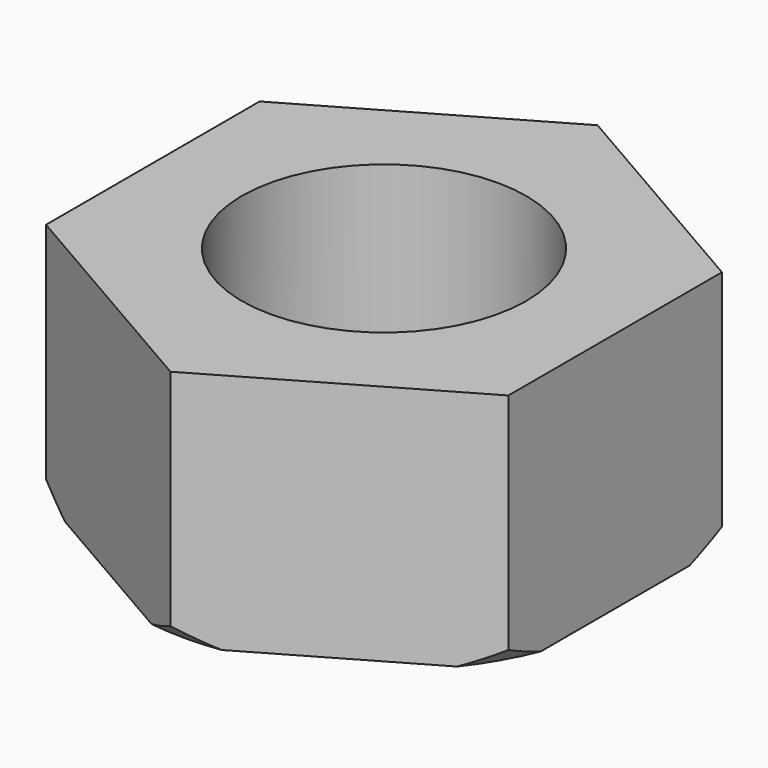
from build123d import *

# Parameters (mm, degrees)
F0_R     = 4
F1_DEPTH = 6.8


with BuildPart() as f1:
    # F0 (on Top) → F1 (new body)
    with BuildSketch(Plane.XY):
        Polygon((-6.5, 3.7527767497), (-6.5, -3.7527767497), (0, -7.5055534995), (6.5, -3.7527767497), (6.5, 3.7527767497), (0, 7.5055534995), align=None)
        Circle(F0_R, mode=Mode.SUBTRACT)
    extrude(amount=F1_DEPTH)

    # F2 (on Right) → F3 (revolve, cut)
    with BuildSketch(Plane.YZ):
        Polygon((7.0055534995, 0), (7.5055534995, 0), (7.5055534995, 0.5), align=None)
    revolve(axis=Axis((0, 0, 0), (0, 0, -1)), mode=Mode.SUBTRACT)


solid = f1.part
